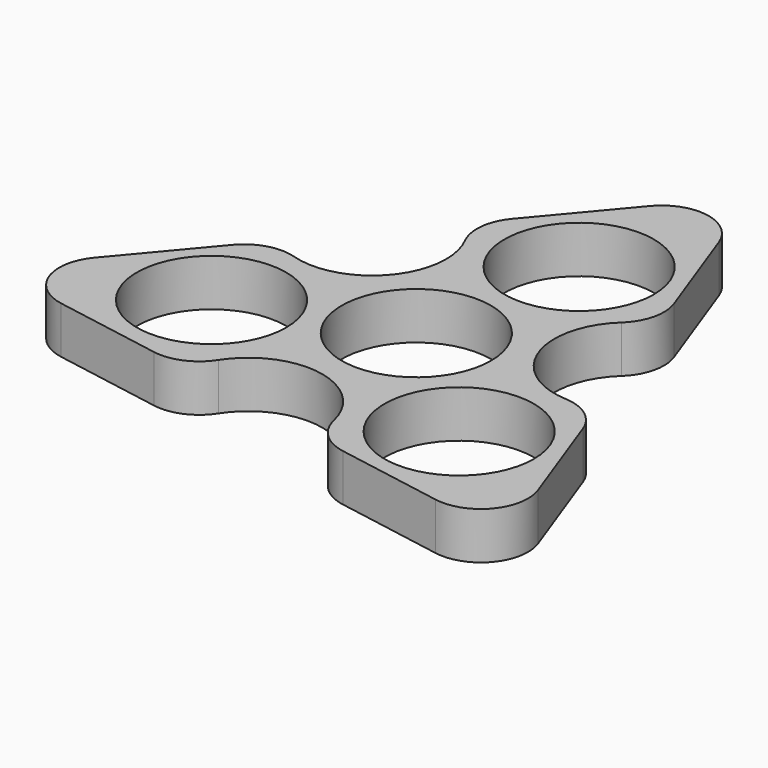
from build123d import *

# Parameters (mm, degrees)
F0_R     = 11.1
F1_DEPTH = 7
F2_R     = 7


with BuildPart() as f1:
    # F0 (on Top) → F1 (new body)
    with BuildSketch(Plane.XY):
        with BuildLine():
            Line((-38.9624627261, -8.1840724655), (-60.7952496686, -34.2480210213))
            Line((-60.7952496686, -34.2480210213), (-27.306814625, -40.123794871))
            ThreePointArc((-27.306814625, -40.123794871), (-15.5182325204, -31.0662352189), (-5.4723209344, -42.0247805283))
            ThreePointArc((-5.4723209344, -42.0247805283), (-5.5137756251, -42.9788689424), (-5.6378272439, -43.9257661855))
            Line((-5.6378272439, -43.9257661855), (27.8506077997, -49.8015400352))
            Line((27.8506077997, -49.8015400352), (16.1949596986, -17.8618176297))
            ThreePointArc((16.1949596986, -17.8618176297), (2.090575123, -11.2993230017), (8.6530697509, 2.8050615739))
            Line((8.6530697509, 2.8050615739), (-3.0025783502, 34.7447839795))
            Line((-3.0025783502, 34.7447839795), (-24.8353652927, 8.6808354236))
            ThreePointArc((-24.8353652927, 8.6808354236), (-21.9314911759, 4.9013893297), (-20.8989140094, 0.2483814791))
            ThreePointArc((-20.8989140094, 0.2483814791), (-27.2459061587, -9.7190413544), (-38.9624627261, -8.1840724655))
        make_face()
        with Locations((-35.7535122499, -24.7765792781)):
            Circle(F0_R, mode=Mode.SUBTRACT)
        with Locations((7.3296251626, -32.6118866408)):
            Circle(F0_R, mode=Mode.SUBTRACT)
        with Locations((-11.9824067397, -16.4349256924)):
            Circle(F0_R, mode=Mode.SUBTRACT)
        with Locations((-7.6287635535, 8.378265008)):
            Circle(F0_R, mode=Mode.SUBTRACT)
    extrude(amount=F1_DEPTH)

    # F2
    f2_edges = [f1.edges().sort_by_distance(p)[0] for p in [
        (-3.002578, 34.744784, 3.5),
        (-24.835365, 8.680835, 3.5),
        (-38.962463, -8.184072, 3.5),
        (-60.79525, -34.248021, 3.5),
        (-27.306815, -40.123795, 3.5),
        (-5.637827, -43.925766, 3.5),
        (16.19496, -17.861818, 3.5),
        (8.65307, 2.805062, 3.5),
        (27.850608, -49.80154, 3.5),
    ]]
    fillet(f2_edges, radius=F2_R)


solid = f1.part
